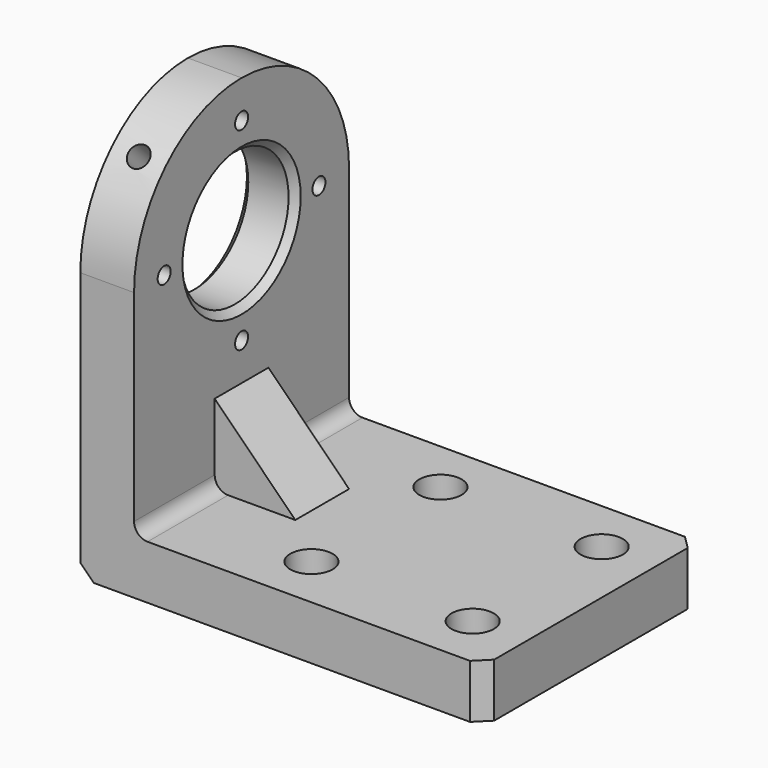
from build123d import *

# Parameters (mm, degrees)
F1_DEPTH        = 100
F2_R            = 99.99999
F3_SIZE         = 10
F5_DEPTH        = 25
F6_R            = 50
F7_DEPTH        = 40.001
F10_D           = 12.1
F11_D           = 15.5
F11_DEPTH       = 70
F11_START       = 0.3007608
F11_TIP         = 4.6566697975
F13_D           = 17.5
F13_CBORE_D     = 31.5
F13_CBORE_DEPTH = 20
F14_SIZE        = 5
F15_R           = 10


# Not quite as in the source:
# - a fillet or chamfer is up to 0.001 mm smaller than in the source, because OpenCascade refuses the exact size


with BuildPart() as f1:
    # F0 (on Front) → F1 (new body, symmetric)
    with BuildSketch(Plane.XZ):
        Polygon((40, 300), (0, 300), (0, 0), (300, 0), (300, 40), (40, 40), align=None)
    extrude(amount=F1_DEPTH, both=True)

    # F2 (radius 100 in the source; OpenCascade refuses exactly that, so slightly less here)
    f2_edges = [f1.edges().sort_by_distance(p)[0] for p in [
        (20, -100, 300),
        (20, 100, 300),
    ]]
    fillet(f2_edges, radius=F2_R)

    # F3
    f3_edges = [f1.edges().sort_by_distance(p)[0] for p in [
        (300, -100, 20),
        (300, 100, 20),
        (0, 0, 0),
    ]]
    chamfer(f3_edges, length=F3_SIZE)

    # F4 (on Front) → F5 (join, symmetric)
    with BuildSketch(Plane.XZ):
        Polygon((40, 100), (40, 40), (100, 40), align=None)
    extrude(amount=F5_DEPTH, both=True)

    # F6 (on face) → F7 (cut, through all)
    with BuildSketch(Plane.YZ.offset(40)):
        with Locations((0, 200)):
            Circle(F6_R)
    extrude(amount=-F7_DEPTH, mode=Mode.SUBTRACT)

    # F10 (through all)
    with Locations(Plane.YZ.offset(40)):
        with Locations((0, 272), (72, 200), (0, 128), (-72, 200)):
            Hole(F10_D / 2)

    # F11
    # its depths count from where the whole tool has entered the part; down to there all is cleared
    with Locations(Plane(origin=(0, -170.7106781187, 170.7106781187), x_dir=(1, 0, 0), z_dir=(0, -0.7071067812, 0.7071067812)).offset(-F11_START)):
        with Locations((20, 141.4213562373)):
            Hole(F11_D / 2, depth=F11_DEPTH)
            with Locations((0, 0, -(F11_DEPTH + F11_TIP / 2))):  # 118° drill point
                Cone(0, F11_D / 2, F11_TIP, mode=Mode.SUBTRACT)

    # F13 (through all)
    with Locations(Plane.XY.offset(40)):
        with Locations((140, -60), (140, 60), (260, 60), (260, -60)):
            CounterBoreHole(F13_D / 2, F13_CBORE_D / 2, F13_CBORE_DEPTH)

    # F14
    f14_edges = [f1.edges().sort_by_distance(p)[0] for p in [
        (40, -50, 200),
        (0, -50, 200),
    ]]
    chamfer(f14_edges, length=F14_SIZE)

    # F15
    f15_edges = [f1.edges().sort_by_distance(p)[0] for p in [
        (40, -62.5, 40),
        (40, 62.5, 40),
    ]]
    fillet(f15_edges, radius=F15_R)


solid = f1.part
